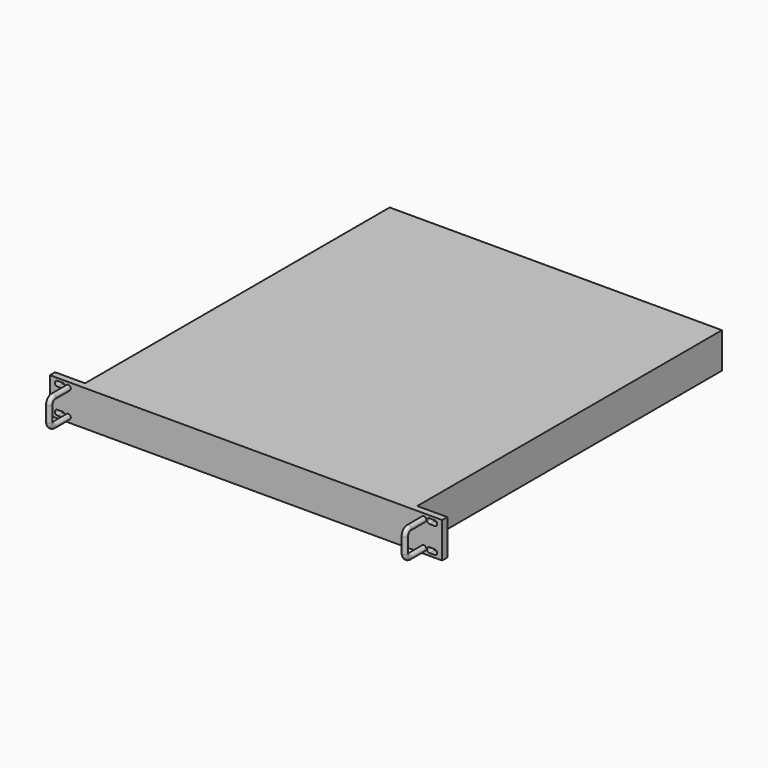
from build123d import *

# Parameters (mm, degrees)
F0_W     = 489.3
F0_H     = 44.5
F1_DEPTH = 483
F2_W     = 37.4
F2_H     = 44.5
F3_DEPTH = 475
F5_DEPTH = 8
F8_R     = 3.175


with BuildPart() as f1:
    # F0 (on Front) → F1 (new body)
    with BuildSketch(Plane.XZ):
        Rectangle(F0_W, F0_H)
    extrude(amount=-F1_DEPTH)

    # F2 (on face) → F3 (cut)
    with BuildSketch(Plane(origin=(0, 483, 0), x_dir=(-1, 0, 0), z_dir=(0, 1, 0))):
        with Locations((-225.95, 0)):
            Rectangle(F2_W, F2_H)
        with Locations((225.95, 0)):
            Rectangle(F2_W, F2_H)
    extrude(amount=-F3_DEPTH, mode=Mode.SUBTRACT)

    # F4 (on face) → F5 (cut, through all)
    with BuildSketch(Plane.XZ):
        with BuildLine():
            Line((-235.325, 12.725), (-228.975, 12.725))
            ThreePointArc((-228.975, 12.725), (-225.8, 15.9), (-228.975, 19.075))
            Line((-228.975, 19.075), (-235.325, 19.075))
            ThreePointArc((-235.325, 19.075), (-238.5, 15.9), (-235.325, 12.725))
        make_face()
        with BuildLine():
            Line((-228.975, -12.725), (-235.325, -12.725))
            ThreePointArc((-235.325, -12.725), (-238.5, -15.9), (-235.325, -19.075))
            Line((-235.325, -19.075), (-228.975, -19.075))
            ThreePointArc((-228.975, -19.075), (-225.8, -15.9), (-228.975, -12.725))
        make_face()
        with BuildLine():
            Line((235.325, 19.075), (228.975, 19.075))
            ThreePointArc((228.975, 19.075), (225.8, 15.9), (228.975, 12.725))
            Line((228.975, 12.725), (235.325, 12.725))
            ThreePointArc((235.325, 12.725), (238.5, 15.9), (235.325, 19.075))
        make_face()
        with BuildLine():
            Line((235.325, -12.725), (228.975, -12.725))
            ThreePointArc((228.975, -12.725), (225.8, -15.9), (228.975, -19.075))
            Line((228.975, -19.075), (235.325, -19.075))
            ThreePointArc((235.325, -19.075), (238.5, -15.9), (235.325, -12.725))
        make_face()
    extrude(amount=-F5_DEPTH, mode=Mode.SUBTRACT)

    # F9: sweep along a path in F7
    with BuildLine(Plane.YZ.offset(-228.6)) as f9_path:
        Line((0, 15.9), (-23.15, 15.9))
        ThreePointArc((-23.15, 15.9), (-27.6401280605, 14.0401280605), (-29.5, 9.55))
        Line((-29.5, 9.55), (-29.5, -9.55))
        ThreePointArc((-29.5, -9.55), (-27.6401280605, -14.0401280605), (-23.15, -15.9))
        Line((-23.15, -15.9), (0, -15.9))
    # F8 (on face) → F9 (sweep)
    with BuildSketch(Plane.XZ):
        with Locations((-221.79, 15.9)):
            Circle(F8_R)
    sweep(path=f9_path.line)

    # F10: F1 across plane


with BuildPart() as f1_1:
    add(f1.part)
    add(f1.part.mirror(Plane.YZ))


solid = f1_1.part
